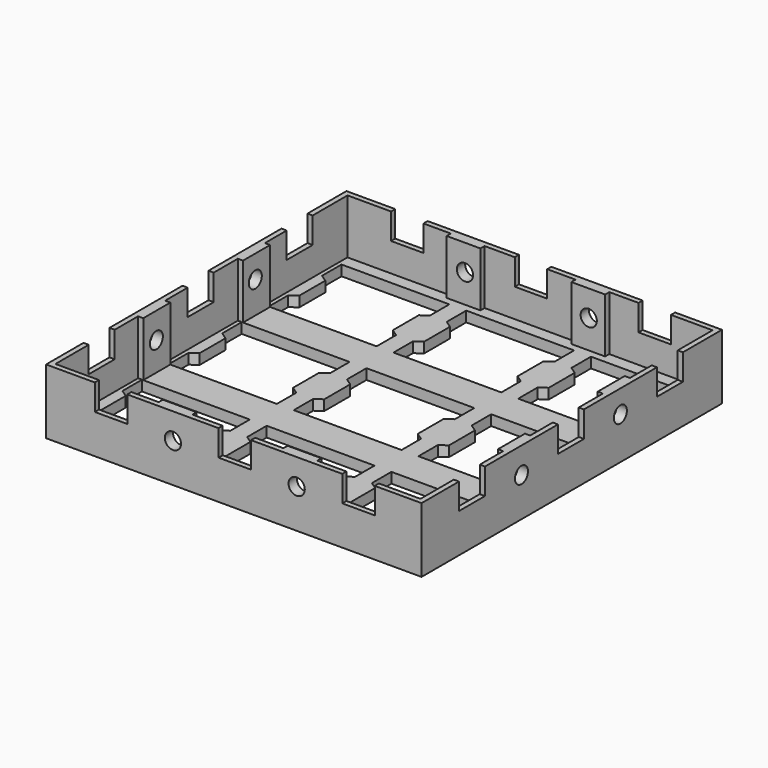
from build123d import *

# Parameters (mm, degrees)
F0_W     = 1.4
F0_H     = 2.7
F1_DEPTH = 1.6
F2_W     = 5.2
F2_H     = 0.8
F2_W_2   = 2.6
F3_DEPTH = 8.4
F2_W_3   = 0.8
F2_H_2   = 5
F2_H_3   = 2.5
F2_H_4   = 2.35
F2_W_4   = 5
F2_W_5   = 2.35
F2_W_6   = 2.65
F2_W_7   = 2.5
F2_H_5   = 2.65
F4_DEPTH = 4.4
F5_R     = 1.25
F6_DEPTH = 57.801
F7_R     = 1.25
F8_DEPTH = 57.801


# Not quite as in the source:
# - a feature names something its author has since deleted; it is built from what else it names


with BuildPart() as f1:
    # F0 (on Top) → F1 (new body)
    with BuildSketch(Plane.XY):
        Polygon((-1.4, 0), (-1.4, 2.7), (0, 2.7), (0, 57.8), (-1.4, 57.8), (-57.8, 57.8), (-57.8, 2.7), (-57.8, 0), align=None)
        Polygon((-39.8, 2.7), (-56.4, 2.7), (-56.4, 6.45), (-56.4, 12.95), (-56.4, 16.7), (-39.8, 16.7), (-39.8, 12.95), (-39.8, 6.45), align=None, mode=Mode.SUBTRACT)
        Polygon((-37.2, 16.7), (-20.6, 16.7), (-20.6, 12.95), (-20.6, 6.45), (-20.6, 2.7), (-37.2, 2.7), (-37.2, 6.45), (-37.2, 12.95), align=None, mode=Mode.SUBTRACT)
        Polygon((-1.4, 6.45), (-1.4, 2.7), (-9.7, 2.7), (-18, 2.7), (-18, 6.45), (-18, 12.95), (-18, 16.7), (-9.7, 16.7), (-1.4, 16.7), (-1.4, 12.95), align=None, mode=Mode.SUBTRACT)
        Polygon((-39.55, 32.0178743874), (-39.8, 31.8474198419), (-39.8, 25.9525801581), (-39.55, 25.7821256126), (-39.55, 21.65), (-56.65, 21.65), (-56.65, 25.7821256126), (-56.4, 25.9525801581), (-56.4, 31.8474198419), (-56.65, 32.0178743874), (-56.65, 36.15), (-39.55, 36.15), align=None, mode=Mode.SUBTRACT)
        Polygon((-20.6, 31.8474198419), (-20.6, 25.9525801581), (-20.35, 25.7821256126), (-20.35, 21.65), (-37.45, 21.65), (-37.45, 25.7821256126), (-37.2, 25.9525801581), (-37.2, 31.8474198419), (-37.45, 32.0178743874), (-37.45, 36.15), (-20.35, 36.15), (-20.35, 32.0178743874), align=None, mode=Mode.SUBTRACT)
        Polygon((-39.8, 55.1), (-39.8, 51.35), (-39.8, 44.85), (-39.8, 41.1), (-56.4, 41.1), (-56.4, 44.85), (-56.4, 51.35), (-56.4, 55.1), align=None, mode=Mode.SUBTRACT)
        Polygon((-20.6, 51.35), (-20.6, 44.85), (-20.6, 41.1), (-37.2, 41.1), (-37.2, 44.85), (-37.2, 51.35), (-37.2, 55.1), (-20.6, 55.1), align=None, mode=Mode.SUBTRACT)
        Polygon((-1.15, 32.0178743874), (-1.4, 31.8474198419), (-1.4, 25.9525801581), (-1.15, 25.7821256126), (-1.15, 21.65), (-18.25, 21.65), (-18.25, 25.7821256126), (-18, 25.9525801581), (-18, 31.8474198419), (-18.25, 32.0178743874), (-18.25, 36.15), (-1.15, 36.15), align=None, mode=Mode.SUBTRACT)
        Polygon((-18, 55.1), (-1.4, 55.1), (-1.4, 51.35), (-1.4, 44.85), (-1.4, 41.1), (-18, 41.1), (-18, 44.85), (-18, 51.35), align=None, mode=Mode.SUBTRACT)
        Polygon((-36.1, 12.2), (-37.2, 12.95), (-37.2, 6.45), (-36.1, 7.2), align=None)
        Polygon((-40.9, 7.2), (-39.8, 6.45), (-39.8, 12.95), (-40.9, 12.2), align=None)
        Polygon((-18, 12.95), (-18, 6.45), (-16.9, 7.2), (-16.9, 12.2), align=None)
        Polygon((-20.6, 6.45), (-20.6, 12.95), (-21.7, 12.2), (-21.7, 7.2), align=None)
        Polygon((-37.2, 51.35), (-37.2, 44.85), (-36.1, 45.6), (-36.1, 50.6), align=None)
        Polygon((-1.4, 44.85), (-1.4, 51.35), (-2.5, 50.6), (-2.5, 45.6), align=None)
        Polygon((-2.5, 7.2), (-1.4, 6.45), (-1.4, 12.95), (-2.5, 12.2), align=None)
        Polygon((-56.4, 12.95), (-56.4, 6.45), (-55.3, 7.2), (-55.3, 12.2), align=None)
        Polygon((-16.9, 50.6), (-18, 51.35), (-18, 44.85), (-16.9, 45.6), align=None)
        Polygon((-21.7, 45.6), (-20.6, 44.85), (-20.6, 51.35), (-21.7, 50.6), align=None)
        Polygon((-39.8, 44.85), (-39.8, 51.35), (-40.9, 50.6), (-40.9, 45.6), align=None)
        Polygon((-55.3, 50.6), (-56.4, 51.35), (-56.4, 44.85), (-55.3, 45.6), align=None)
        Polygon((-39.8, 35.9), (-39.8, 32.15), (-39.8, 31.8474198419), (-39.55, 32.0178743874), (-39.55, 36.15), (-56.65, 36.15), (-56.65, 32.0178743874), (-56.4, 31.8474198419), (-56.4, 32.15), (-56.4, 35.9), align=None)
        Polygon((-39.55, 25.7821256126), (-39.8, 25.9525801581), (-39.8, 25.65), (-39.8, 21.9), (-56.4, 21.9), (-56.4, 25.65), (-56.4, 25.9525801581), (-56.65, 25.7821256126), (-56.65, 21.65), (-39.55, 21.65), align=None)
        Polygon((-20.6, 32.15), (-20.6, 31.8474198419), (-20.35, 32.0178743874), (-20.35, 36.15), (-37.45, 36.15), (-37.45, 32.0178743874), (-37.2, 31.8474198419), (-37.2, 32.15), (-37.2, 35.9), (-20.6, 35.9), align=None)
        Polygon((-20.6, 25.9525801581), (-20.6, 25.65), (-20.6, 21.9), (-37.2, 21.9), (-37.2, 25.65), (-37.2, 25.9525801581), (-37.45, 25.7821256126), (-37.45, 21.65), (-20.35, 21.65), (-20.35, 25.7821256126), align=None)
        Polygon((-18, 35.9), (-1.4, 35.9), (-1.4, 32.15), (-1.4, 31.8474198419), (-1.15, 32.0178743874), (-1.15, 36.15), (-18.25, 36.15), (-18.25, 32.0178743874), (-18, 31.8474198419), (-18, 32.15), align=None)
        Polygon((-1.15, 25.7821256126), (-1.4, 25.9525801581), (-1.4, 25.65), (-1.4, 21.9), (-18, 21.9), (-18, 25.65), (-18, 25.9525801581), (-18.25, 25.7821256126), (-18.25, 21.65), (-1.15, 21.65), align=None)
        Polygon((-55.55, 31.2678743874), (-56.4, 31.8474198419), (-56.4, 25.9525801581), (-55.55, 26.5321256126), align=None)
        Polygon((-39.8, 25.9525801581), (-39.8, 31.8474198419), (-40.65, 31.2678743874), (-40.65, 26.5321256126), align=None)
        Polygon((-37.2, 31.8474198419), (-37.2, 25.9525801581), (-36.35, 26.5321256126), (-36.35, 31.2678743874), align=None)
        Polygon((-21.45, 26.5321256126), (-20.6, 25.9525801581), (-20.6, 31.8474198419), (-21.45, 31.2678743874), align=None)
        Polygon((-17.15, 31.2678743874), (-18, 31.8474198419), (-18, 25.9525801581), (-17.15, 26.5321256126), align=None)
        Polygon((-1.4, 25.9525801581), (-1.4, 31.8474198419), (-2.25, 31.2678743874), (-2.25, 26.5321256126), align=None)
        with Locations((-0.7, 1.35)):
            Rectangle(F0_W, F0_H)
        Polygon((-55.3, 31.4), (-56.4, 32.15), (-56.4, 31.8474198419), (-55.55, 31.2678743874), (-55.55, 26.5321256126), (-56.4, 25.9525801581), (-56.4, 25.65), (-55.3, 26.4), align=None)
        Polygon((-39.8, 31.8474198419), (-39.8, 32.15), (-40.9, 31.4), (-40.9, 26.4), (-39.8, 25.65), (-39.8, 25.9525801581), (-40.65, 26.5321256126), (-40.65, 31.2678743874), align=None)
        Polygon((-37.2, 25.9525801581), (-37.2, 25.65), (-36.1, 26.4), (-36.1, 31.4), (-37.2, 32.15), (-37.2, 31.8474198419), (-36.35, 31.2678743874), (-36.35, 26.5321256126), align=None)
        Polygon((-21.7, 26.4), (-20.6, 25.65), (-20.6, 25.9525801581), (-21.45, 26.5321256126), (-21.45, 31.2678743874), (-20.6, 31.8474198419), (-20.6, 32.15), (-21.7, 31.4), align=None)
        Polygon((-16.9, 31.4), (-18, 32.15), (-18, 31.8474198419), (-17.15, 31.2678743874), (-17.15, 26.5321256126), (-18, 25.9525801581), (-18, 25.65), (-16.9, 26.4), align=None)
        Polygon((-1.4, 31.8474198419), (-1.4, 32.15), (-2.5, 31.4), (-2.5, 26.4), (-1.4, 25.65), (-1.4, 25.9525801581), (-2.25, 26.5321256126), (-2.25, 31.2678743874), align=None)
    extrude(amount=F1_DEPTH)

    # F2 (on face) → F3 (join)
    with BuildSketch(Plane.XY.offset(1.6)):
        Polygon((-12.2, 57), (-12.2, 57.8), (-26.25, 57.8), (-26.25, 57), (-21.9, 57), (-16.7, 57), align=None)
        Polygon((-31.25, 57), (-31.25, 57.8), (-45.3, 57.8), (-45.3, 57), (-41.1, 57), (-35.9, 57), align=None)
        Polygon((-26.25, 0), (-12.2, 0), (-12.2, 0.8), (-16.7, 0.8), (-19.3, 0.8), (-21.9, 0.8), (-26.25, 0.8), align=None)
        Polygon((-45.3, 0), (-31.25, 0), (-31.25, 0.8), (-35.9, 0.8), (-38.5, 0.8), (-41.1, 0.8), (-45.3, 0.8), align=None)
        Polygon((-57.8, 26.25), (-57.8, 12.2), (-57, 12.2), (-57, 16.7), (-57, 21.9), (-57, 26.25), align=None)
        Polygon((-57.8, 45.3), (-57.8, 31.25), (-57, 31.25), (-57, 35.9), (-57, 41.1), (-57, 45.3), align=None)
        Polygon((-0.8, 31.25), (0, 31.25), (0, 45.3), (-0.8, 45.3), (-0.8, 41.1), (-0.8, 35.9), align=None)
        Polygon((-0.8, 12.2), (0, 12.2), (0, 26.25), (-0.8, 26.25), (-0.8, 21.9), (-0.8, 16.7), align=None)
        Polygon((-57.8, 57.8), (-57.8, 50.3), (-57, 50.3), (-57, 57), (-50.3, 57), (-50.3, 57.8), align=None)
        Polygon((-0.8, 50.3), (0, 50.3), (0, 57.8), (-7.2, 57.8), (-7.2, 57), (-0.8, 57), align=None)
        Polygon((-7.2, 0), (0, 0), (0, 7.2), (-0.8, 7.2), (-0.8, 0.8), (-7.2, 0.8), align=None)
        Polygon((-57.8, 0), (-50.3, 0), (-50.3, 0.8), (-57, 0.8), (-57, 7.2), (-57.8, 7.2), align=None)
        with Locations((-38.5, 56.6)):
            Rectangle(F2_W, F2_H)
        with Locations((-19.3, 56.6)):
            Rectangle(F2_W, F2_H)
        with Locations((-39.8, 1.2)):
            Rectangle(F2_W_2, F2_H)
        with Locations((-37.2, 1.2)):
            Rectangle(F2_W_2, F2_H)
        with Locations((-20.6, 1.2)):
            Rectangle(F2_W_2, F2_H)
        with Locations((-18, 1.2)):
            Rectangle(F2_W_2, F2_H)
        Polygon((-57, 41.1), (-57, 35.9), (-56.4, 35.9), (-56.2, 35.9), (-56.2, 41.1), (-56.4, 41.1), align=None)
        Polygon((-57, 21.9), (-57, 16.7), (-56.4, 16.7), (-56.2, 16.7), (-56.2, 21.9), (-56.4, 21.9), align=None)
        Polygon((-1.4, 35.9), (-0.8, 35.9), (-0.8, 41.1), (-1.4, 41.1), (-1.6, 41.1), (-1.6, 35.9), align=None)
        Polygon((-1.4, 16.7), (-0.8, 16.7), (-0.8, 21.9), (-1.4, 21.9), (-1.6, 21.9), (-1.6, 16.7), align=None)
    extrude(amount=F3_DEPTH)

    # F2 (on face) → F4 (join)
    with BuildSketch(Plane.XY.offset(1.6)):
        with Locations((-57.4, 47.8)):
            Rectangle(F2_W_3, F2_H_2)
        with Locations((-57.4, 28.75)):
            Rectangle(F2_W_3, F2_H_2)
        with Locations((-57.4, 9.7)):
            Rectangle(F2_W_3, F2_H_2)
        with Locations((-0.4, 10.95)):
            Rectangle(F2_W_3, F2_H_3)
        with Locations((-0.4, 8.45)):
            Rectangle(F2_W_3, F2_H_3)
        with Locations((-0.4, 30.075)):
            Rectangle(F2_W_3, F2_H_4)
        with Locations((-0.4, 47.8)):
            Rectangle(F2_W_3, F2_H_2)
        with Locations((-47.8, 57.4)):
            Rectangle(F2_W_4, F2_H)
        with Locations((-28.75, 57.4)):
            Rectangle(F2_W_4, F2_H)
        with Locations((-9.7, 57.4)):
            Rectangle(F2_W_4, F2_H)
        with Locations((-47.8, 0.4)):
            Rectangle(F2_W_4, F2_H)
        with Locations((-30.075, 0.4)):
            Rectangle(F2_W_5, F2_H)
        with Locations((-27.575, 0.4)):
            Rectangle(F2_W_6, F2_H)
        with Locations((-8.45, 0.4)):
            Rectangle(F2_W_7, F2_H)
        with Locations((-10.95, 0.4)):
            Rectangle(F2_W_7, F2_H)
        with Locations((-0.4, 27.575)):
            Rectangle(F2_W_3, F2_H_5)
    extrude(amount=F4_DEPTH)

    # F5 (on face) → F6 (cut, through all)
    with BuildSketch(Plane(origin=(-57.8, 0, 0), x_dir=(0, -1, 0), z_dir=(-1, 0, 0))):
        with Locations((-38.2631011868, 6.4759525297)):
            Circle(F5_R)
        with BuildLine():
            Line((-19.225, 6), (-17.975, 6))
            ThreePointArc((-17.975, 6), (-19.225, 7.25), (-20.475, 6))
            Line((-20.475, 6), (-19.225, 6))
        make_face()
        with BuildLine():
            ThreePointArc((-20.475, 6), (-19.225, 4.75), (-17.975, 6))
            Line((-17.975, 6), (-19.225, 6))
            Line((-19.225, 6), (-20.475, 6))
        make_face()
    extrude(amount=-F6_DEPTH, mode=Mode.SUBTRACT)

    # F7 (on face) → F8 (cut, through all)
    with BuildSketch(Plane.XZ):
        with BuildLine():
            Line((-19.225, 6), (-17.975, 6))
            ThreePointArc((-17.975, 6), (-19.225, 7.25), (-20.475, 6))
            Line((-20.475, 6), (-19.225, 6))
        make_face()
        with BuildLine():
            ThreePointArc((-20.475, 6), (-19.225, 4.75), (-17.975, 6))
            Line((-17.975, 6), (-19.225, 6))
            Line((-19.225, 6), (-20.475, 6))
        make_face()
        with Locations((-38.275, 6)):
            Circle(F7_R)
    extrude(amount=-F8_DEPTH, mode=Mode.SUBTRACT)


solid = f1.part
